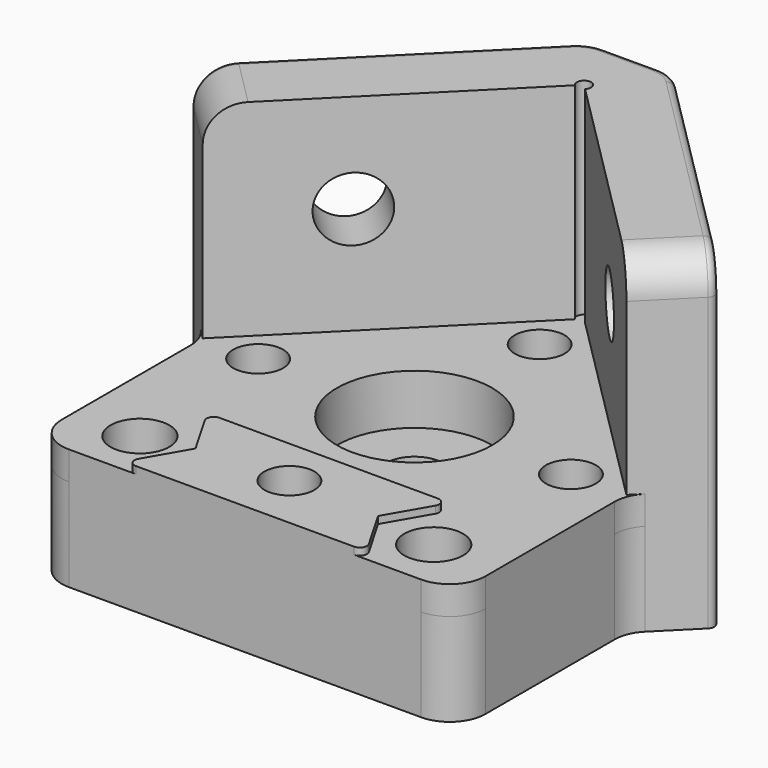
from build123d import *

# Parameters (mm, degrees)
F0_R          = 4.125
F0_R_2        = 1.7
F0_R_3        = 4.05
F1_DEPTH      = 13
F3_DEPTH      = 45.87
F4_R          = 4.5
F5_DEPTH      = 10
F6_R          = 4.25
F7_DEPTH      = 10
F8_R          = 7
F9_DEPTH      = 3
F10_R         = 7
F11_DEPTH     = 3
F13_R         = 5
F12_R         = 3.5
F14_DEPTH     = 2.9
F15_TEXT_SIZE = 7.1642815932
F16_DEPTH     = 0.25
F17_R         = 3.5
F18_DEPTH     = 5
F19_T1_DEPTH  = 43.37
F19_T3_DEPTH  = 9.3301270189
F19_T5_DEPTH  = 36.6690475583
F19_T7_DEPTH  = 7.5391052434
F19_T9_DEPTH  = 36.6690475583
F19_T12_ANGLE = 90
F19_T14_ANGLE = 45
F19_T16_ANGLE = 45
F19_T18_ANGLE = 90
F20_R         = 1
F21_DEPTH     = 32.87
F24_DEPTH     = 4
F25_R         = 10.875
F26_DEPTH     = 7.05
F29_R         = 4.125
F29_R_2       = 1.7
F29_R_3       = 4.05
F30_DEPTH     = 17
F31_R         = 3.5
F32_DEPTH     = 5


# Not quite as in the source:
# - a fillet or chamfer that OpenCascade refuses, or shapes differently, is made with other operations: its cross-section is extruded or revolved along the edge and cut away or added
# - a feature names something its author has since deleted; it is built from what else it names
# - Text() gives the source's letters only with a copy of the font that has no kerning and outlines rounded to 1/6400 em; it was checked with that copy


with BuildPart() as f1:
    # F0 (on Top) → F1 (new body)
    with BuildSketch(Plane.XY):
        Polygon((-29.6984848098, 0), (0, 0), (29.6984848098, 0), (29.6984848098, 29.7), (0, 59.3984848098), (-29.6984848098, 29.7), align=None)
        with Locations((-20.59, 7.3196897832)):
            Circle(F0_R, mode=Mode.SUBTRACT)
        with Locations((0, 7.7796897832)):
            Circle(F0_R_2, mode=Mode.SUBTRACT)
        with Locations((20.59, 7.3196897832)):
            Circle(F0_R, mode=Mode.SUBTRACT)
        with Locations((-21.9203102168, 29.7)):
            Circle(F0_R_2, mode=Mode.SUBTRACT)
        with Locations((0, 29.7)):
            Circle(F0_R_3, mode=Mode.SUBTRACT)
        with Locations((21.9203102168, 29.7)):
            Circle(F0_R_2, mode=Mode.SUBTRACT)
        with Locations((0, 51.6203102168)):
            Circle(F0_R_2, mode=Mode.SUBTRACT)
    extrude(amount=F1_DEPTH)

    # F2 (on face) → F3 (join)
    with BuildSketch(Plane(origin=(0, 0, 0), x_dir=(1, 0, 0), z_dir=(0, 0, -1))):
        Polygon((0, -59.3984848098), (-29.6984848098, -29.7), (-36.7695526217, -36.7710678119), (-5.8406204336, -67.7), (0, -67.7), (5.8406204336, -67.7), (36.7695526217, -36.7710678119), (29.6984848098, -29.7), align=None)
    extrude(amount=-F3_DEPTH)

    # F4 (on face) → F5 (cut, through all)
    with BuildSketch(Plane(origin=(-29.6992424049, 29.6992424049, 0), x_dir=(0.7071067812, 0.7071067812, 0), z_dir=(0.7071067812, -0.7071067812, 0))):
        with Locations((16.6010714012, 32)):
            Circle(F4_R)
    extrude(amount=-F5_DEPTH, mode=Mode.SUBTRACT)

    # F6 (on face) → F7 (cut, through all)
    with BuildSketch(Plane(origin=(29.6992424049, 29.6992424049, 0), x_dir=(0.7071067812, -0.7071067812, 0), z_dir=(-0.7071067812, -0.7071067812, 0))):
        with Locations((-16.6010714012, 32)):
            Circle(F6_R)
    extrude(amount=-F7_DEPTH, mode=Mode.SUBTRACT)

    # F8 (on face) → F9 (cut)
    with BuildSketch(Plane(origin=(-36.7703102168, 36.7703102168, 0), x_dir=(-0.7071067812, -0.7071067812, 0), z_dir=(-0.7071067812, 0.7071067812, 0))):
        with Locations((-16.6010714005, 32)):
            Circle(F8_R)
    extrude(amount=-F9_DEPTH, mode=Mode.SUBTRACT)

    # F10 (on face) → F11 (cut)
    with BuildSketch(Plane(origin=(36.7703102168, 36.7703102168, 0), x_dir=(-0.7071067812, 0.7071067812, 0), z_dir=(0.7071067812, 0.7071067812, 0))):
        with Locations((16.6010714007, 32)):
            Circle(F10_R)
    extrude(amount=-F11_DEPTH, mode=Mode.SUBTRACT)

    # F13
    f13_edges = [f1.edges().sort_by_distance(p)[0] for p in [
        (33.234019, 33.235534, 45.87),
        (-33.234019, 33.235534, 45.87),
        (29.698485, 29.7, 6.5),
        (29.698485, 0, 6.5),
        (-29.698485, 0, 6.5),
        (-29.698485, 29.7, 6.5),
        (-5.84062, 67.7, 22.935),
        (5.84062, 67.7, 22.935),
    ]]
    fillet(f13_edges, radius=F13_R)

    # F12 (on face) → F14 (cut)
    with BuildSketch(Plane.XY.offset(13)):
        with Locations((0, 51.6203102168)):
            Circle(F12_R)
        with Locations((-21.9203102168, 29.7)):
            Circle(F12_R)
        with Locations((21.9203102168, 29.7)):
            Circle(F12_R)
        with Locations((0, 7.7796897832)):
            Circle(F12_R)
    extrude(amount=-F14_DEPTH, mode=Mode.SUBTRACT)

    # F15 (on face) → F16 (cut)
    with BuildSketch(Plane(origin=(-36.7703102168, 36.7703102168, 0), x_dir=(-0.7071067812, -0.7071067812, 0), z_dir=(-0.7071067812, 0.7071067812, 0))):
        with Locations((-41.6701189596, 3.2)):
            Text('SIENCI LABS', F15_TEXT_SIZE, font='Open Sans', text_align=(TextAlign.LEFT, TextAlign.BOTTOM))
    extrude(amount=-F16_DEPTH, mode=Mode.SUBTRACT)

    # F17 (on face) → F18 (join)
    with BuildSketch(Plane.XY.offset(13)):
        Polygon((16.692885683, 14.0696897832), (-16.692885683, 14.0696897832), (-12.7957713659, 7.3196897832), (-16.692885683, 0.5696897832), (16.692885683, 0.5696897832), (12.7957713659, 7.3196897832), align=None)
        with Locations((0, 7.7796897832)):
            Circle(F17_R, mode=Mode.SUBTRACT)
        Polygon((16.692885683, 0.5696897832), (-16.692885683, 0.5696897832), (-17.0217962327, 0), (0, 0), (17.0217962327, 0), align=None)
        Polygon((-17.0217962327, 14.6393795664), (-16.692885683, 14.0696897832), (16.692885683, 14.0696897832), (17.0217962327, 14.6393795664), (0, 14.6393795664), align=None)
    extrude(amount=F18_DEPTH)

    # F19: fillet of radius 1 on 13 edges, made by hand

    # F19_s2 → F19_t1 (cut)
    with BuildSketch(Plane.XY.offset(-2.5)):
        with BuildLine():
            ThreePointArc((36.0624458405, 37.4781745931), (36.3553390593, 36.7710678119), (36.0624458405, 36.0639610307))
            Line((36.0624458405, 36.0639610307), (36.7695526217, 36.7710678119))
            Line((36.7695526217, 36.7710678119), (36.0624458405, 37.4781745931))
        make_face()
        with BuildLine():
            ThreePointArc((-36.0624458405, 36.0639610307), (-36.3553390593, 36.7710678119), (-36.0624458405, 37.4781745931))
            Line((-36.0624458405, 37.4781745931), (-36.7695526217, 36.7710678119))
            Line((-36.7695526217, 36.7710678119), (-36.0624458405, 36.0639610307))
        make_face()
    extrude(amount=F19_T1_DEPTH, mode=Mode.SUBTRACT)

    # F19_s4 → F19_t3 (cut)
    with BuildSketch(Plane.XY.offset(13)):
        with BuildLine():
            ThreePointArc((-15.2897454251, 0), (-16.1557708289, 0.5), (-16.1557708289, 1.5))
            Line((-16.1557708289, 1.5), (-17.0217962327, 0))
            Line((-17.0217962327, 0), (-15.2897454251, 0))
        make_face()
        with BuildLine():
            ThreePointArc((-15.2897454251, 14.6393795664), (-16.1557708289, 14.1393795664), (-16.1557708289, 13.1393795664))
            Line((-16.1557708289, 13.1393795664), (-17.0217962327, 14.6393795664))
            Line((-17.0217962327, 14.6393795664), (-15.2897454251, 14.6393795664))
        make_face()
        with BuildLine():
            ThreePointArc((16.1557708289, 13.1393795664), (16.1557708289, 14.1393795664), (15.2897454251, 14.6393795664))
            Line((15.2897454251, 14.6393795664), (17.0217962327, 14.6393795664))
            Line((17.0217962327, 14.6393795664), (16.1557708289, 13.1393795664))
        make_face()
        with BuildLine():
            ThreePointArc((15.2897454251, 0), (16.1557708289, 0.5), (16.1557708289, 1.5))
            Line((16.1557708289, 1.5), (17.0217962327, 0))
            Line((17.0217962327, 0), (15.2897454251, 0))
        make_face()
    extrude(amount=F19_T3_DEPTH, mode=Mode.SUBTRACT)

    # F19_s6 → F19_t5 (cut)
    with BuildSketch(Plane(origin=(3.536291501, 3.536291501, 0), x_dir=(0, 0, 1), z_dir=(0.7071067812, 0.7071067812, 0))):
        with BuildLine():
            ThreePointArc((44.87, -52.0010714012), (45.5771067812, -51.7081781824), (45.87, -51.0010714012))
            Line((45.87, -51.0010714012), (45.87, -52.0010714012))
            Line((45.87, -52.0010714012), (44.87, -52.0010714012))
        make_face()
    extrude(amount=F19_T5_DEPTH, mode=Mode.SUBTRACT)

    # F19_s8 → F19_t7 (cut)
    with BuildSketch(Plane.YZ.offset(-3.7695526217)):
        with BuildLine():
            ThreePointArc((67.7, 44.87), (67.4071067812, 45.5771067812), (66.7, 45.87))
            Line((66.7, 45.87), (67.7, 45.87))
            Line((67.7, 45.87), (67.7, 44.87))
        make_face()
    extrude(amount=F19_T7_DEPTH, mode=Mode.SUBTRACT)

    # F19_s10 → F19_t9 (cut)
    with BuildSketch(Plane(origin=(-29.4652236891, 29.4652236891, 0), x_dir=(0, 0, 1), z_dir=(0.7071067812, -0.7071067812, 0))):
        with BuildLine():
            ThreePointArc((44.87, -52.0010714012), (45.5771067812, -51.7081781824), (45.87, -51.0010714012))
            Line((45.87, -51.0010714012), (45.87, -52.0010714012))
            Line((45.87, -52.0010714012), (44.87, -52.0010714012))
        make_face()
    extrude(amount=F19_T9_DEPTH, mode=Mode.SUBTRACT)

    # F19_s11 → F19_t12 (revolve, cut)
    with BuildSketch(Plane.XY.offset(40.87)):
        with BuildLine():
            ThreePointArc((-36.0624458405, 37.4781745931), (-36.3553390593, 36.7710678119), (-36.0624458405, 36.0639610307))
            Line((-36.0624458405, 36.0639610307), (-36.7695526217, 36.7710678119))
            Line((-36.7695526217, 36.7710678119), (-36.0624458405, 37.4781745931))
        make_face()
    revolve(axis=Axis((-33.2340187158, 40.3066017178, 40.87), (-0.7071067812, 0.7071067812, 0)), revolution_arc=F19_T12_ANGLE, mode=Mode.SUBTRACT)

    # F19_s13 → F19_t14 (revolve, cut)
    with BuildSketch(Plane.YZ.offset(-3.7695526217)):
        with BuildLine():
            ThreePointArc((67.7, 44.87), (67.4071067812, 45.5771067812), (66.7, 45.87))
            Line((66.7, 45.87), (67.7, 45.87))
            Line((67.7, 45.87), (67.7, 44.87))
        make_face()
    revolve(axis=Axis((-3.7695526217, 62.7, 45.87), (0, 0, 1)), revolution_arc=F19_T14_ANGLE, mode=Mode.SUBTRACT)

    # F19_s15 → F19_t16 (revolve, cut)
    with BuildSketch(Plane(origin=(-29.4652236891, 29.4652236891, 0), x_dir=(0, 0, 1), z_dir=(0.7071067812, -0.7071067812, 0))):
        with BuildLine():
            ThreePointArc((44.87, -52.0010714012), (45.5771067812, -51.7081781824), (45.87, -51.0010714012))
            Line((45.87, -51.0010714012), (45.87, -52.0010714012))
            Line((45.87, -52.0010714012), (44.87, -52.0010714012))
        make_face()
    revolve(axis=Axis((3.7695526217, 62.7, 45.87), (0, 0, 1)), revolution_arc=F19_T16_ANGLE, mode=Mode.SUBTRACT)

    # F19_s17 → F19_t18 (revolve, cut)
    with BuildSketch(Plane.XY.offset(40.87)):
        with BuildLine():
            ThreePointArc((36.0624458405, 37.4781745931), (36.3553390593, 36.7710678119), (36.0624458405, 36.0639610307))
            Line((36.0624458405, 36.0639610307), (36.7695526217, 36.7710678119))
            Line((36.7695526217, 36.7710678119), (36.0624458405, 37.4781745931))
        make_face()
    revolve(axis=Axis((33.2340187158, 40.3066017178, 40.87), (-0.7071067812, -0.7071067812, 0)), revolution_arc=F19_T18_ANGLE, mode=Mode.SUBTRACT)

    # F20 (on face) → F21 (cut, through all)
    with BuildSketch(Plane.XY.offset(45.87)):
        with Locations((0, 59.3984848098)):
            Circle(F20_R)
    extrude(amount=-F21_DEPTH, mode=Mode.SUBTRACT)

    # F23 (on face) → F24 (join)
    with BuildSketch(Plane.XY.offset(13)):
        with BuildLine():
            Line((31.1629509039, 31.1644660941), (29.6984848098, 29.7))
            Line((29.6984848098, 29.7), (0.7071067812, 58.6913780286))
            ThreePointArc((0.7071067812, 58.6913780286), (0, 60.3984848098), (-0.7071067812, 58.6913780286))
            Line((-0.7071067812, 58.6913780286), (-29.6984848098, 29.7))
            Line((-29.6984848098, 29.7), (-31.1629509039, 31.1644660941))
            ThreePointArc((-31.1629509039, 31.1644660941), (-30.0790871473, 29.54234935), (-29.6984848098, 27.6289321881))
            Line((-29.6984848098, 27.6289321881), (-29.6984848098, 5))
            ThreePointArc((-29.6984848098, 5), (-28.2340187158, 1.4644660941), (-24.6984848098, 0))
            Line((-24.6984848098, 0), (-15.2897454251, 0))
            ThreePointArc((-15.2897454251, 0), (-16.1557708289, 0.5), (-16.1557708289, 1.5))
            Line((-16.1557708289, 1.5), (-12.7957713659, 7.3196897832))
            Line((-12.7957713659, 7.3196897832), (-16.1557708289, 13.1393795664))
            ThreePointArc((-16.1557708289, 13.1393795664), (-16.1557708289, 14.1393795664), (-15.2897454251, 14.6393795664))
            Line((-15.2897454251, 14.6393795664), (15.2897454251, 14.6393795664))
            ThreePointArc((15.2897454251, 14.6393795664), (16.1557708289, 14.1393795664), (16.1557708289, 13.1393795664))
            Line((16.1557708289, 13.1393795664), (12.7957713659, 7.3196897832))
            Line((12.7957713659, 7.3196897832), (16.1557708289, 1.5))
            ThreePointArc((16.1557708289, 1.5), (16.1557708289, 0.5), (15.2897454251, 0))
            Line((15.2897454251, 0), (24.6984848098, 0))
            ThreePointArc((24.6984848098, 0), (28.2340187158, 1.4644660941), (29.6984848098, 5))
            Line((29.6984848098, 5), (29.6984848098, 27.6289321881))
            ThreePointArc((29.6984848098, 27.6289321881), (30.0790871473, 29.54234935), (31.1629509039, 31.1644660941))
        make_face()
    extrude(amount=F24_DEPTH)

    # F25 (on face) → F26 (cut)
    with BuildSketch(Plane.XY.offset(17)):
        with Locations((0, 29.7)):
            Circle(F25_R)
    extrude(amount=-F26_DEPTH, mode=Mode.SUBTRACT)

    # F29 (on face) → F30 (cut, through all)
    with BuildSketch(Plane.XY.offset(17)):
        with Locations((-20.59, 7.3196897832)):
            Circle(F29_R)
        with Locations((20.59, 7.3196897832)):
            Circle(F29_R)
        with Locations((0, 7.7796897832)):
            Circle(F29_R_2)
        with Locations((-21.9203102168, 29.7)):
            Circle(F29_R_2)
        with Locations((0, 51.6203102168)):
            Circle(F29_R_2)
        with Locations((0, 29.7)):
            Circle(F29_R_3)
        with Locations((21.9203102168, 29.7)):
            Circle(F29_R_2)
    extrude(amount=-F30_DEPTH, mode=Mode.SUBTRACT)

    # F31 (on face) → F32 (cut)
    with BuildSketch(Plane.XY.offset(17)):
        with Locations((-21.9203102168, 29.7)):
            Circle(F31_R)
        with Locations((21.9203102168, 29.7)):
            Circle(F31_R)
        with Locations((0, 51.6203102168)):
            Circle(F31_R)
        with Locations((0, 7.7796897832)):
            Circle(F31_R)
    extrude(amount=-F32_DEPTH, mode=Mode.SUBTRACT)


solid = f1.part
